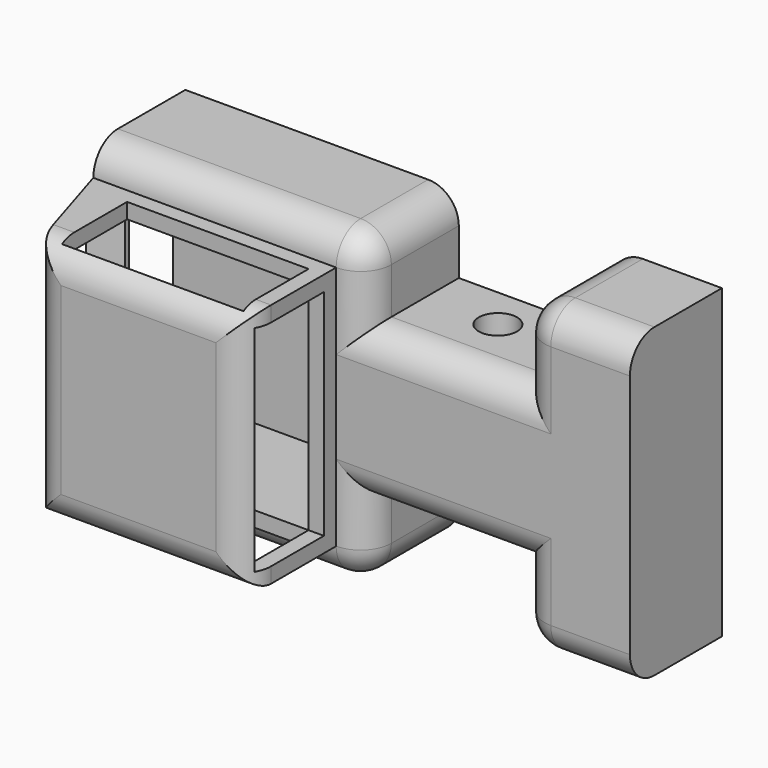
from build123d import *

# Parameters (mm, degrees)
F0_W         = 88.9
F0_H         = 25.4
F1_DEPTH     = 19.05
F2_W         = 25.4
F2_H         = 19.05
F3_DEPTH     = 12.7
F4_R         = 3.175
F5_DEPTH     = 12.7
F7_R         = 5.08
F8_W         = 37.6902104366
F8_H         = 35.56
F9_DEPTH     = 16.51
F10_W        = 40.2302104366
F10_H        = 40.64
F11_DEPTH    = 18.55363
F12_W        = 31.75
F12_H        = 35.56
F13_DEPTH    = 16.51
F14_W        = 30.0702104366
F14_H        = 13.47363
F15_DEPTH    = 2.54
F16_W        = 30.0702104366
F16_H        = 13.47363
F17_DEPTH    = 2.54
F19_DEPTH    = 50.8
F20_W        = 14.3303479189
F20_H        = 35.56
F21_DEPTH    = 7.62
F22_W        = 13.47363
F22_H        = 35.56
F23_DEPTH    = 5.08
F24_T1_DEPTH = 59.4053934524
F24_T3_DEPTH = 59.927191924
F24_T5_DEPTH = 66.04


# Not quite as in the source:
# - a fillet or chamfer that OpenCascade refuses, or shapes differently, is made with other operations: its cross-section is extruded or revolved along the edge and cut away or added


with BuildPart() as f1:
    # F0 (on Front) → F1 (new body)
    with BuildSketch(Plane.XZ):
        with Locations((44.45, 12.7)):
            Rectangle(F0_W, F0_H)
    extrude(amount=F1_DEPTH)

    # F2 (on face) → F3 (cut)
    with BuildSketch(Plane.XY.offset(25.4)):
        with Locations((58.0102104366, -9.525)):
            Rectangle(F2_W, F2_H)
    extrude(amount=-F3_DEPTH, mode=Mode.SUBTRACT)

    # F4 (on face) → F5 (cut)
    with BuildSketch(Plane.XY.offset(12.7)):
        with Locations((57.3752104366, -6.985)):
            Circle(F4_R)
    extrude(amount=-F5_DEPTH, mode=Mode.SUBTRACT)

    # F6: F1 across plane


with BuildPart() as f1_1:
    add(f1.part)
    add(f1.part.mirror(Plane.XY))

    # F7
    f7_edges = [f1_1.edges().sort_by_distance(p)[0] for p in [
        (22.655105, -19.05, -25.4),
        (22.655105, -19.05, 25.4),
        (45.31021, -9.525, -25.4),
        (45.31021, -19.05, -19.05),
        (70.71021, -19.05, -19.05),
        (70.71021, -9.525, -25.4),
        (70.71021, -9.525, 25.4),
        (70.71021, -19.05, 19.05),
        (45.31021, -9.525, 25.4),
        (45.31021, -19.05, 19.05),
        (58.01021, -19.05, -12.7),
        (58.01021, -19.05, 12.7),
        (79.805105, -19.05, -25.4),
        (79.805105, -19.05, 25.4),
    ]]
    fillet(f7_edges, radius=F7_R)

    # F8 (on face) → F9 (cut)
    with BuildSketch(Plane.XZ.offset(19.05)):
        with Locations((18.8451052183, 0)):
            Rectangle(F8_W, F8_H)
    extrude(amount=-F9_DEPTH, mode=Mode.SUBTRACT)

    # F10 (on face) → F11 (join)
    with BuildSketch(Plane.XZ.offset(19.05)):
        with Locations((20.1151052183, 0)):
            Rectangle(F10_W, F10_H)
    extrude(amount=F11_DEPTH)

    # F12 (on face) → F13 (cut)
    with BuildSketch(Plane(origin=(0, -19.05, 0), x_dir=(-1, 0, 0), z_dir=(0, 1, 0))):
        with Locations((-21.8152104366, 0)):
            Rectangle(F12_W, F12_H)
    extrude(amount=-F13_DEPTH, mode=Mode.SUBTRACT)

    # F14 (on face) → F15 (cut)
    with BuildSketch(Plane(origin=(0, 0, -20.32), x_dir=(1, 0, 0), z_dir=(0, 0, -1))):
        with Locations((22.6551052183, 28.326815)):
            Rectangle(F14_W, F14_H)
    extrude(amount=-F15_DEPTH, mode=Mode.SUBTRACT)

    # F16 (on face) → F17 (cut)
    with BuildSketch(Plane.XY.offset(20.32)):
        with Locations((22.6551052183, -28.326815)):
            Rectangle(F16_W, F16_H)
    extrude(amount=-F17_DEPTH, mode=Mode.SUBTRACT)

    # F18 (on face) → F19 (cut)
    with BuildSketch(Plane.XY.offset(20.32)):
        Polygon((0, -37.60363), (5.7030185126, -37.60363), (0, -19.05), align=None)
    extrude(amount=-F19_DEPTH, mode=Mode.SUBTRACT)

    # F20 (on face) → F21 (cut)
    with BuildSketch(Plane(origin=(-5.3501013979, -1.6445152413, 0), x_dir=(0.293813307, -0.9558628252, 0), z_dir=(-0.9558628252, -0.293813307, 0))):
        with Locations((27.9143607796, 0)):
            Rectangle(F20_W, F20_H)
    extrude(amount=-F21_DEPTH, mode=Mode.SUBTRACT)

    # F22 (on face) → F23 (cut)
    with BuildSketch(Plane.YZ.offset(40.2302104366)):
        with Locations((-28.326815, 0)):
            Rectangle(F22_W, F22_H)
    extrude(amount=-F23_DEPTH, mode=Mode.SUBTRACT)

    # F24: fillet of radius 5.08 on 4 edges, made by hand

    # F24_s2 → F24_t1 (cut)
    with BuildSketch(Plane.XY.offset(-29.7026967262)):
        with BuildLine():
            ThreePointArc((9.4560972031, -37.60363), (6.4374769658, -36.6094997805), (4.600314051, -34.0162015997))
            Line((4.600314051, -34.0162015997), (5.7030185126, -37.60363))
            Line((5.7030185126, -37.60363), (9.4560972031, -37.60363))
        make_face()
    extrude(amount=F24_T1_DEPTH, mode=Mode.SUBTRACT)

    # F24_s4 → F24_t3 (cut)
    with BuildSketch(Plane.YZ.offset(-6.9969814874)):
        with BuildLine():
            ThreePointArc((-37.60363, 15.24), (-36.1157324484, 18.8321024484), (-32.52363, 20.32))
            Line((-32.52363, 20.32), (-37.60363, 20.32))
            Line((-37.60363, 20.32), (-37.60363, 15.24))
        make_face()
        with BuildLine():
            ThreePointArc((-37.60363, -15.24), (-36.1157324484, -18.8321024484), (-32.52363, -20.32))
            Line((-32.52363, -20.32), (-37.60363, -20.32))
            Line((-37.60363, -20.32), (-37.60363, -15.24))
        make_face()
    extrude(amount=F24_T3_DEPTH, mode=Mode.SUBTRACT)

    # F24_s6 → F24_t5 (cut)
    with BuildSketch(Plane.XY.offset(-33.02)):
        with BuildLine():
            ThreePointArc((40.2302104366, -32.52363), (38.742312885, -36.1157324484), (35.1502104366, -37.60363))
            Line((35.1502104366, -37.60363), (40.2302104366, -37.60363))
            Line((40.2302104366, -37.60363), (40.2302104366, -32.52363))
        make_face()
    extrude(amount=F24_T5_DEPTH, mode=Mode.SUBTRACT)


solid = f1_1.part
